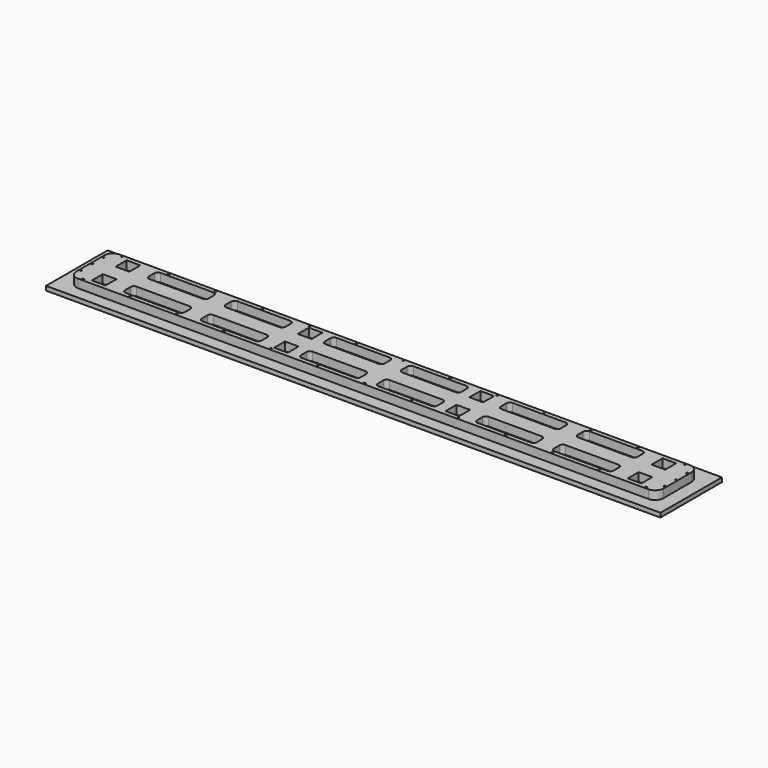
from build123d import *

# Parameters (mm, degrees)
F0_W     = 874.014
F0_H     = 77.5716
F0_W_2   = 2.9972
F0_H_2   = 0.9906
F0_W_3   = 20.32
F0_H_3   = 20.32
F0_W_4   = 0.9906
F0_H_4   = 2.9972
F0_W_5   = 88.9
F1_DEPTH = 12.7
F2_W     = 914.4
F2_H     = 114.3
F3_DEPTH = 6.35
F4_R     = 12.7
F5_R     = 5.08
F6_R     = 5.08


with BuildPart() as f1:
    # F0 (on Top) → F1 (new body)
    with BuildSketch(Plane.XY):
        Rectangle(F0_W, F0_H)
        with Locations((-419.1, -35.9029)):
            Rectangle(F0_W_2, F0_H_2, mode=Mode.SUBTRACT)
        with Locations((-349.25, -35.9029)):
            Rectangle(F0_W_2, F0_H_2, mode=Mode.SUBTRACT)
        with Locations((-279.4, -35.9029)):
            Rectangle(F0_W_2, F0_H_2, mode=Mode.SUBTRACT)
        with Locations((-398.78, -22.225)):
            Rectangle(F0_W_3, F0_H_3, mode=Mode.SUBTRACT)
        with Locations((-434.1114, -20.8788)):
            Rectangle(F0_W_4, F0_H_4, mode=Mode.SUBTRACT)
        with Locations((-319.1074297856, -22.225)):
            Rectangle(F0_W_5, F0_H_3, mode=Mode.SUBTRACT)
        with Locations((-209.55, -35.9029)):
            Rectangle(F0_W_2, F0_H_2, mode=Mode.SUBTRACT)
        with Locations((-139.7, -35.9029)):
            Rectangle(F0_W_2, F0_H_2, mode=Mode.SUBTRACT)
        with Locations((-69.85, -35.9029)):
            Rectangle(F0_W_2, F0_H_2, mode=Mode.SUBTRACT)
        with Locations((0, -35.9029)):
            Rectangle(F0_W_2, F0_H_2, mode=Mode.SUBTRACT)
        with Locations((-204.8074297856, -22.225)):
            Rectangle(F0_W_5, F0_H_3, mode=Mode.SUBTRACT)
        with Locations((-127.635, -22.225)):
            Rectangle(F0_W_3, F0_H_3, mode=Mode.SUBTRACT)
        with Locations((-57.15, -22.225)):
            Rectangle(F0_W_5, F0_H_3, mode=Mode.SUBTRACT)
        with Locations((69.85, -35.9029)):
            Rectangle(F0_W_2, F0_H_2, mode=Mode.SUBTRACT)
        with Locations((139.7, -35.9029)):
            Rectangle(F0_W_2, F0_H_2, mode=Mode.SUBTRACT)
        with Locations((209.55, -35.9029)):
            Rectangle(F0_W_2, F0_H_2, mode=Mode.SUBTRACT)
        with Locations((57.15, -22.225)):
            Rectangle(F0_W_5, F0_H_3, mode=Mode.SUBTRACT)
        with Locations((127.635, -22.225)):
            Rectangle(F0_W_3, F0_H_3, mode=Mode.SUBTRACT)
        with Locations((204.8074297856, -22.225)):
            Rectangle(F0_W_5, F0_H_3, mode=Mode.SUBTRACT)
        with Locations((279.4, -35.9029)):
            Rectangle(F0_W_2, F0_H_2, mode=Mode.SUBTRACT)
        with Locations((349.25, -35.9029)):
            Rectangle(F0_W_2, F0_H_2, mode=Mode.SUBTRACT)
        with Locations((419.1, -35.9029)):
            Rectangle(F0_W_2, F0_H_2, mode=Mode.SUBTRACT)
        with Locations((319.1074297856, -22.225)):
            Rectangle(F0_W_5, F0_H_3, mode=Mode.SUBTRACT)
        with Locations((398.78, -22.225)):
            Rectangle(F0_W_3, F0_H_3, mode=Mode.SUBTRACT)
        with Locations((434.1114, -20.8788)):
            Rectangle(F0_W_4, F0_H_4, mode=Mode.SUBTRACT)
        with Locations((-434.1114, 0)):
            Rectangle(F0_W_4, F0_H_4, mode=Mode.SUBTRACT)
        with Locations((-434.1114, 20.8788)):
            Rectangle(F0_W_4, F0_H_4, mode=Mode.SUBTRACT)
        with Locations((-398.78, 22.225)):
            Rectangle(F0_W_3, F0_H_3, mode=Mode.SUBTRACT)
        with Locations((-319.1074297856, 22.225)):
            Rectangle(F0_W_5, F0_H_3, mode=Mode.SUBTRACT)
        with Locations((-419.1, 35.9029)):
            Rectangle(F0_W_2, F0_H_2, mode=Mode.SUBTRACT)
        with Locations((-349.25, 35.9029)):
            Rectangle(F0_W_2, F0_H_2, mode=Mode.SUBTRACT)
        with Locations((-279.4, 35.9029)):
            Rectangle(F0_W_2, F0_H_2, mode=Mode.SUBTRACT)
        with Locations((-204.8074297856, 22.225)):
            Rectangle(F0_W_5, F0_H_3, mode=Mode.SUBTRACT)
        with Locations((-127.635, 22.225)):
            Rectangle(F0_W_3, F0_H_3, mode=Mode.SUBTRACT)
        with Locations((-57.15, 22.225)):
            Rectangle(F0_W_5, F0_H_3, mode=Mode.SUBTRACT)
        with Locations((-209.55, 35.9029)):
            Rectangle(F0_W_2, F0_H_2, mode=Mode.SUBTRACT)
        with Locations((-139.7, 35.9029)):
            Rectangle(F0_W_2, F0_H_2, mode=Mode.SUBTRACT)
        with Locations((-69.85, 35.9029)):
            Rectangle(F0_W_2, F0_H_2, mode=Mode.SUBTRACT)
        with Locations((0, 35.9029)):
            Rectangle(F0_W_2, F0_H_2, mode=Mode.SUBTRACT)
        with Locations((434.1114, 0)):
            Rectangle(F0_W_4, F0_H_4, mode=Mode.SUBTRACT)
        with Locations((57.15, 22.225)):
            Rectangle(F0_W_5, F0_H_3, mode=Mode.SUBTRACT)
        with Locations((127.635, 22.225)):
            Rectangle(F0_W_3, F0_H_3, mode=Mode.SUBTRACT)
        with Locations((204.8074297856, 22.225)):
            Rectangle(F0_W_5, F0_H_3, mode=Mode.SUBTRACT)
        with Locations((69.85, 35.9029)):
            Rectangle(F0_W_2, F0_H_2, mode=Mode.SUBTRACT)
        with Locations((139.7, 35.9029)):
            Rectangle(F0_W_2, F0_H_2, mode=Mode.SUBTRACT)
        with Locations((209.55, 35.9029)):
            Rectangle(F0_W_2, F0_H_2, mode=Mode.SUBTRACT)
        with Locations((319.1074297856, 22.225)):
            Rectangle(F0_W_5, F0_H_3, mode=Mode.SUBTRACT)
        with Locations((434.1114, 20.8788)):
            Rectangle(F0_W_4, F0_H_4, mode=Mode.SUBTRACT)
        with Locations((398.78, 22.225)):
            Rectangle(F0_W_3, F0_H_3, mode=Mode.SUBTRACT)
        with Locations((279.4, 35.9029)):
            Rectangle(F0_W_2, F0_H_2, mode=Mode.SUBTRACT)
        with Locations((349.25, 35.9029)):
            Rectangle(F0_W_2, F0_H_2, mode=Mode.SUBTRACT)
        with Locations((419.1, 35.9029)):
            Rectangle(F0_W_2, F0_H_2, mode=Mode.SUBTRACT)
    extrude(amount=F1_DEPTH)

    # F4
    f4_edges = [f1.edges().sort_by_distance(p)[0] for p in [
        (-437.007, 38.7858, 6.35),
        (-437.007, -38.7858, 6.35),
        (437.007, 38.7858, 6.35),
        (437.007, -38.7858, 6.35),
    ]]
    fillet(f4_edges, radius=F4_R)

    # F5
    f5_edges = [f1.edges().sort_by_distance(p)[0] for p in [
        (363.55743, -12.065, 6.35),
        (249.25743, -12.065, 6.35),
        (249.25743, 32.385, 6.35),
        (363.55743, 32.385, 6.35),
        (101.6, -12.065, 6.35),
        (101.6, 32.385, 6.35),
        (-12.7, -12.065, 6.35),
        (-12.7, 32.385, 6.35),
        (-160.35743, -12.065, 6.35),
        (-160.35743, 32.385, 6.35),
        (-274.65743, 32.385, 6.35),
        (-274.65743, -12.065, 6.35),
        (-363.55743, -32.385, 6.35),
        (-363.55743, 12.065, 6.35),
        (-249.25743, 12.065, 6.35),
        (-249.25743, -32.385, 6.35),
        (-101.6, 12.065, 6.35),
        (-101.6, -32.385, 6.35),
        (160.35743, -32.385, 6.35),
        (12.7, -32.385, 6.35),
        (12.7, 32.385, 6.35),
        (-101.6, 32.385, 6.35),
        (-249.25743, 32.385, 6.35),
        (-249.25743, -12.065, 6.35),
        (-363.55743, -12.065, 6.35),
        (-363.55743, 32.385, 6.35),
        (-160.35743, 12.065, 6.35),
        (-12.7, -32.385, 6.35),
        (-12.7, 12.065, 6.35),
        (160.35743, -12.065, 6.35),
        (12.7, -12.065, 6.35),
        (-101.6, -12.065, 6.35),
        (274.65743, -12.065, 6.35),
        (274.65743, 32.385, 6.35),
        (160.35743, 32.385, 6.35),
        (363.55743, 12.065, 6.35),
        (363.55743, -32.385, 6.35),
        (249.25743, -32.385, 6.35),
        (249.25743, 12.065, 6.35),
        (101.6, -32.385, 6.35),
        (274.65743, -32.385, 6.35),
        (274.65743, 12.065, 6.35),
        (-274.65743, 12.065, 6.35),
        (-274.65743, -32.385, 6.35),
        (12.7, 12.065, 6.35),
        (160.35743, 12.065, 6.35),
    ]]
    fillet(f5_edges, radius=F5_R)

    # F6
    f6_edges = [f1.edges().sort_by_distance(p)[0] for p in [
        (-160.35743, -32.385, 6.35),
        (101.6, 12.065, 6.35),
    ]]
    fillet(f6_edges, radius=F6_R)


with BuildPart() as f3:
    # F2 (on face) → F3 (new body)
    with BuildSketch(Plane(origin=(0, 0, 0), x_dir=(1, 0, 0), z_dir=(0, 0, -1))):
        Rectangle(F2_W, F2_H)
    extrude(amount=F3_DEPTH)


solid = Compound([f1.part, f3.part])
